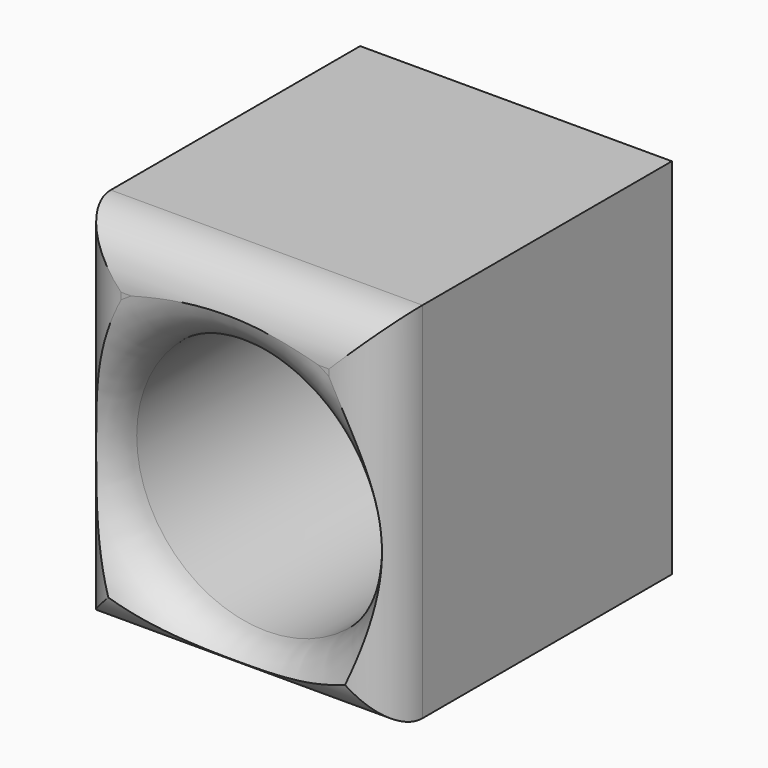
from build123d import *

# Parameters (mm, degrees)
F0_W        = 30
F0_H        = 30
F0_R        = 12.5
F1_DEPTH    = 17.5
F2_DEPTH    = 5
F3_T1_DEPTH = 55
F3_T3_DEPTH = 60


# Not quite as in the source:
# - a fillet or chamfer that OpenCascade refuses, or shapes differently, is made with other operations: its cross-section is extruded or revolved along the edge and cut away or added


with BuildPart() as f1:
    # F0 (on Front) → F1 (new body, symmetric)
    with BuildSketch(Plane.XZ):
        Rectangle(F0_W, F0_H)
        Circle(F0_R, mode=Mode.SUBTRACT)
    extrude(amount=F1_DEPTH, both=True)

    # F2 (add): a face of the model
    f2_faces = [f1.faces().sort_by_distance(p)[0] for p in [
        (0, 0, 15),
    ]]
    extrude(f2_faces, amount=F2_DEPTH)

    # F3: fillet of radius 5 on 5 edges, made by hand

    # F3_s2 → F3_t1 (cut)
    with BuildSketch(Plane.YZ.offset(-27.5)):
        with BuildLine():
            ThreePointArc((-12.5, -15), (-16.0355339059, -13.5355339059), (-17.5, -10))
            Line((-17.5, -10), (-17.5, -15))
            Line((-17.5, -15), (-12.5, -15))
        make_face()
        with BuildLine():
            ThreePointArc((-17.5, 15), (-16.0355339059, 18.5355339059), (-12.5, 20))
            Line((-12.5, 20), (-17.5, 20))
            Line((-17.5, 20), (-17.5, 15))
        make_face()
    extrude(amount=F3_T1_DEPTH, mode=Mode.SUBTRACT)

    # F3_s4 → F3_t3 (cut)
    with BuildSketch(Plane.XY.offset(-27.5)):
        with BuildLine():
            ThreePointArc((15, -12.5), (13.5355339059, -16.0355339059), (10, -17.5))
            Line((10, -17.5), (15, -17.5))
            Line((15, -17.5), (15, -12.5))
        make_face()
        with BuildLine():
            ThreePointArc((-15, -12.5), (-13.5355339059, -16.0355339059), (-10, -17.5))
            Line((-10, -17.5), (-15, -17.5))
            Line((-15, -17.5), (-15, -12.5))
        make_face()
    extrude(amount=F3_T3_DEPTH, mode=Mode.SUBTRACT)

    # F3_s5 → F3_t6 (revolve, cut)
    with BuildSketch(Plane.XY):
        with BuildLine():
            ThreePointArc((17.5, -17.5), (13.9644660941, -16.0355339059), (12.5, -12.5))
            Line((12.5, -12.5), (12.5, -17.5))
            Line((12.5, -17.5), (17.5, -17.5))
        make_face()
    revolve(axis=Axis((0, -17.5, 0), (0, -1, 0)), mode=Mode.SUBTRACT)


solid = f1.part
